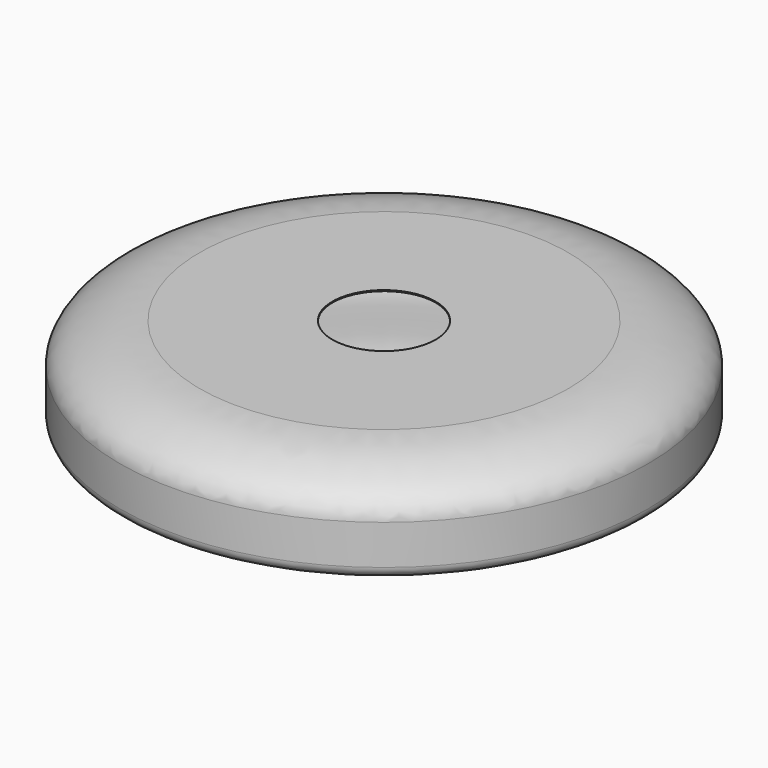
from build123d import *

# Parameters (mm, degrees)
F5_COPIES_COUNT = 50


# Not quite as in the source:
# - a pattern or mirror of a feature is missing from the dataset's text; its kind, count and spacing are read off the source's solid


with BuildPart() as f1:
    # F0 (on Front) → F1 (revolve)
    with BuildSketch(Plane.XZ):
        with BuildLine():
            add(Edge.make_bspline(
                [(116.853825748, 0.5235271343), (141.0117149353, 0), (168.275, -10.8879250748), (168.275, -25.5833492609)],
                knots=[0, 0, 0, 0, 57.6689358023, 57.6689358023, 57.6689358023, 57.6689358023], degree=3))
            Line((168.275, -25.5833492609), (168.275, -48.4433492609))
            add(Edge.make_bspline(
                [(168.275, -48.4433492609), (168.1913842005, -57.0671034475), (136.800647626, -67.4007038792), (41.2932177606, -43.8415680986), (25.277559705, -128.4196608336), (0, -94.7264728657)],
                knots=[0, 0, 0, 0, 0.2444586046, 0.6733079565, 1, 1, 1, 1], degree=3))
            Line((0, -94.7264728657), (0, -95.3614728657))
            add(Edge.make_bspline(
                [(0, -95.3614728657), (25.277559705, -128.8817822517), (41.4936958774, -45.2751496862), (136.4080011868, -68.291392256), (168.8377912523, -57.1846863926), (168.91, -49.911980704)],
                knots=[0, 0, 0, 0, 0.3259861706, 0.7547270609, 1, 1, 1, 1], degree=3))
            Line((168.91, -49.911980704), (168.91, -24.511980704))
            add(Edge.make_bspline(
                [(168.91, -24.511980704), (168.91, -9.7573771756), (140.8997029066, 1.1585271343), (117.8836673498, 1.1585271343)],
                knots=[0, 0, 0, 0, 57.1197128529, 57.1197128529, 57.1197128529, 57.1197128529], degree=3))
            Line((117.8836673498, 1.1585271343), (33.02, 1.1585271343))
            Line((33.02, 1.1585271343), (33.02, 0.5235271343))
            Line((33.02, 0.5235271343), (116.853825748, 0.5235271343))
        make_face()
    revolve(axis=Axis((0, 0, -47.6807364329), (0, 0, -1)))

    # F4 (on face) → F5 (join, up to the next surface of F1)
    with BuildSketch(Plane(origin=(-107.7630734528, -107.7630734528, 0), x_dir=(0.7071067812, -0.7071067812, 0), z_dir=(-0.7071067812, -0.7071067812, 0))):
        with BuildLine():
            add(Edge.make_bspline(
                [(71.806074389, -39.4999235868), (71.5646540911, -47.6975520405), (72.5949747162, -51.4410332824), (63.4895045581, -55.3561263385), (52.8522965393, -57.3901794851)],
                knots=[0, 0, 0, 0, 0.4401357027, 1, 1, 1, 1], degree=3))
            Line((71.806074389, -39.4999235868), (71.1371566841, -39.4999235868))
            ThreePointArc((71.1371566841, -39.4999235868), (67.4416529048, -41.0942885203), (66.0658269354, -44.8765960998))
            add(Edge.make_bspline(
                [(66.0658269354, -44.8765960998), (66.171727548, -46.6868646744), (66.7689525826, -51.3972943975), (60.8864146443, -51.2559585148), (57.3228179978, -51.6866156404)],
                knots=[0.2470779886, 0.2470779886, 0.2470779886, 0.2470779886, 0.46732984, 0.8354827954, 0.8354827954, 0.8354827954, 0.8354827954], degree=3))
            ThreePointArc((57.3228179978, -51.6866156404), (54.130813211, -53.3601851267), (52.8522965393, -56.7299216897))
            Line((52.8522965393, -56.7299216897), (52.8522965393, -57.3901794851))
        make_face()
    f5 = extrude(until=Until.NEXT)

    # F5_copies: F5 ×50 about axis
    f5_copies_axis = Axis((0, 0, 0), (0, 0, 1))
    for i in range(1, F5_COPIES_COUNT):
        add(f5.rotate(f5_copies_axis, i * 360 / F5_COPIES_COUNT))


solid = f1.part
